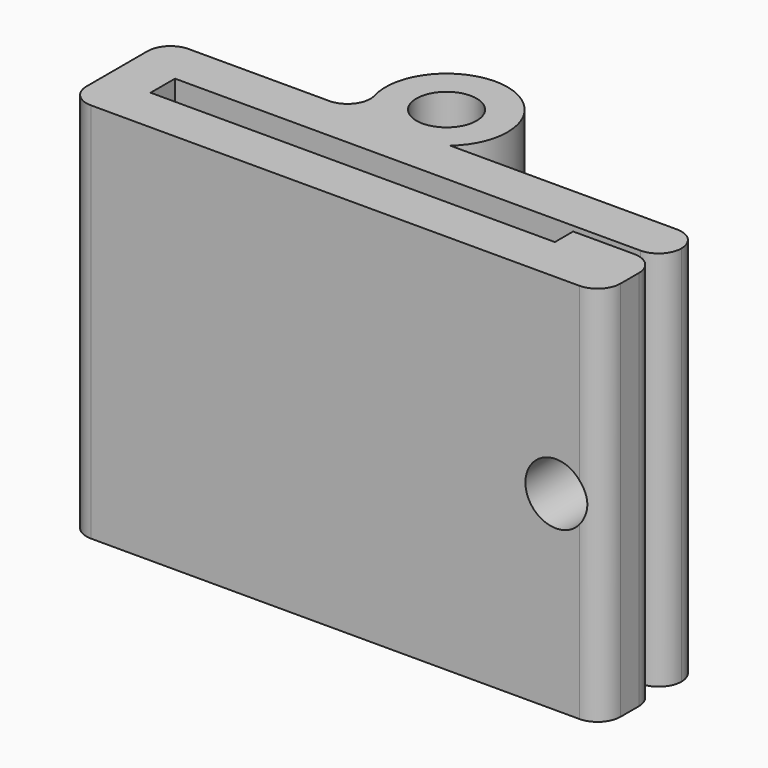
from build123d import *

# Parameters (mm, degrees)
F0_R     = 1.975
F1_DEPTH = 25
F2_R     = 1.49999
F4_DEPTH = 25
F5_DEPTH = 4.8


# Not quite as in the source:
# - a fillet or chamfer is up to 0.001 mm smaller than in the source, because OpenCascade refuses the exact size
# - a feature names something its author has since deleted; it is built from what else it names


with BuildPart() as f1:
    # F0 (on Top) → F1 (new body)
    with BuildSketch(Plane.XY):
        with BuildLine():
            Line((19, 8), (2.6457513111, 8))
            ThreePointArc((2.6457513111, 8), (0, 15), (-2.6457513111, 8))
            Line((-2.6457513111, 8), (-16, 8))
            Line((-16, 8), (-16, 0))
            Line((-16, 0), (19, 0))
            Line((19, 0), (19, 3))
            Line((19, 3), (17.2, 3))
            Line((17.2, 3), (13.5, 3))
            Line((13.5, 3), (-13, 3))
            Line((-13, 3), (-13, 5))
            Line((-13, 5), (19, 5))
            Line((19, 5), (19, 8))
        make_face()
        with Locations((0, 11)):
            Circle(F0_R, mode=Mode.SUBTRACT)
        Polygon((17.2, 3), (19, 3), (19, 4.5), (13.5, 4.5), (13.5, 3), align=None)
    extrude(amount=F1_DEPTH)

    # F2 (radius 1.5 in the source; OpenCascade refuses exactly that, so slightly less here)
    f2_edges = [f1.edges().sort_by_distance(p)[0] for p in [
        (-16, 8, 12.5),
        (-16, 0, 12.5),
        (19, 0, 12.5),
        (19, 5, 12.5),
        (19, 4.5, 12.5),
        (-2.645751, 8, 12.5),
        (19, 8, 12.5),
    ]]
    fillet(f2_edges, radius=F2_R)

    # F3 (on face) → F4 (cut)
    with BuildSketch(Plane.XZ):
        with BuildLine():
            Line((17.50001, 11.6511331714), (17.50001, 13.3488668286))
            ThreePointArc((17.50001, 13.3488668286), (14.2196750343, 12.5), (17.50001, 11.6511331714))
        make_face()
        with BuildLine():
            ThreePointArc((17.7196750343, 12.5), (17.6638689709, 12.9384140794), (17.50001, 13.3488668286))
            Line((17.50001, 13.3488668286), (17.50001, 11.6511331714))
            ThreePointArc((17.50001, 11.6511331714), (17.6638689709, 12.0615859206), (17.7196750343, 12.5))
        make_face()
    extrude(amount=-F4_DEPTH, mode=Mode.SUBTRACT)

    # F3 (on face) → F5 (cut)
    with BuildSketch(Plane.XZ):
        with BuildLine():
            Line((17.50001, 13.3488668286), (17.50001, 13.7876625694))
            ThreePointArc((17.50001, 13.7876625694), (13.9696750343, 12.5), (17.50001, 11.2123374306))
            Line((17.50001, 11.2123374306), (17.50001, 11.6511331714))
            ThreePointArc((17.50001, 11.6511331714), (14.2196750343, 12.5), (17.50001, 13.3488668286))
        make_face()
        with BuildLine():
            ThreePointArc((17.50001, 11.2123374306), (17.8485935971, 11.8146788824), (17.9696750343, 12.5))
            ThreePointArc((17.9696750343, 12.5), (17.8485935971, 13.1853211176), (17.50001, 13.7876625694))
            Line((17.50001, 13.7876625694), (17.50001, 13.3488668286))
            ThreePointArc((17.50001, 13.3488668286), (17.6638689709, 12.9384140794), (17.7196750343, 12.5))
            ThreePointArc((17.7196750343, 12.5), (17.6638689709, 12.0615859206), (17.50001, 11.6511331714))
            Line((17.50001, 11.6511331714), (17.50001, 11.2123374306))
        make_face()
    extrude(amount=-F5_DEPTH, mode=Mode.SUBTRACT)


solid = f1.part
